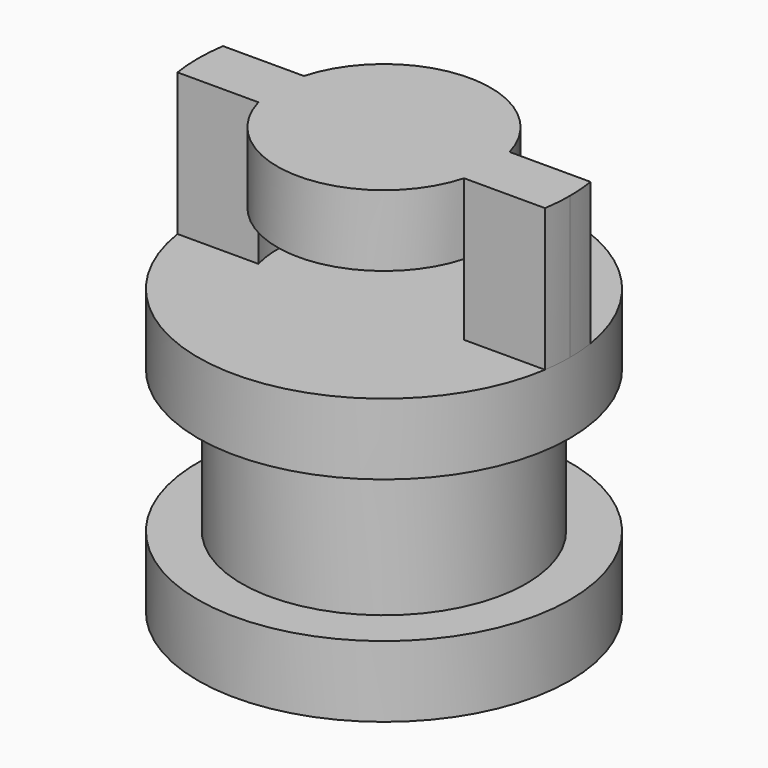
from build123d import *
from build123d import SkipClean  # not in build123d's __all__

# Parameters (mm, degrees)
F0_R      = 4.15
F1_DEPTH  = 1.5875
F3_R      = 4.15
F4_DEPTH  = 1.5875
F6_R      = 2.38125
F7_DEPTH  = 1.5875
F9_DEPTH  = 3.175
F10_R     = 3.175
F11_DEPTH = 3.175
F12_R     = 1.524
F13_DEPTH = 5.159375


# Not quite as in the source:
# - after a boolean that leaves OpenCascade's solid faulty, fix() repairs it


with BuildPart() as f1:
    # F0 (on Top) → F1 (new body)
    with BuildSketch(Plane.XY):
        Circle(F0_R)
    extrude(amount=F1_DEPTH)



with BuildPart() as f4:
    # F3 (on offset) → F4 (new body)
    with BuildSketch(Plane.XY.offset(6.35)):
        Circle(F3_R)
    extrude(amount=-F4_DEPTH)



with BuildPart() as f7:
    # F6 (on offset) → F7 (new body)
    with BuildSketch(Plane.XY.offset(7.9375)):
        Circle(F6_R)
    extrude(amount=F7_DEPTH)


with BuildPart() as f4_1:
    add(f4.part, clean=False)

    add(f7.part)  # F9 merges F7
    # F8 (on face) → F9 (join, through all)
    with BuildSketch(Plane.XY.offset(6.35)):
        with BuildLine():
            Line((2.2950221268, -0.635), (4.1011309416, -0.635))
            ThreePointArc((4.1011309416, -0.635), (4.1377646989, -0.3184388422), (4.15, 0))
            ThreePointArc((4.15, 0), (4.1377646989, 0.3184388422), (4.1011309416, 0.635))
            Line((4.1011309416, 0.635), (2.2950221268, 0.635))
            ThreePointArc((2.2950221268, 0.635), (2.38125, 0), (2.2950221268, -0.635))
        make_face()
        with BuildLine():
            ThreePointArc((-4.1011309416, 0.635), (-4.15, 0), (-4.1011309416, -0.635))
            Line((-4.1011309416, -0.635), (-2.2950221268, -0.635))
            ThreePointArc((-2.2950221268, -0.635), (-2.38125, 0), (-2.2950221268, 0.635))
            Line((-2.2950221268, 0.635), (-4.1011309416, 0.635))
        make_face()
    extrude(amount=F9_DEPTH)

    add(f4_1.part.fix(), mode=Mode.REPLACE)


with BuildPart() as f1_1:
    add(f1.part, clean=False)

    add(f4_1.part)  # F11 merges F4
    # F10 (on face) → F11 (join, through all)
    with BuildSketch(Plane.XY.offset(1.5875)):
        Circle(F10_R)
    extrude(amount=F11_DEPTH)

    # F12 (on face) → F13 (cut)
    with BuildSketch(Plane(origin=(0, 0, 0), x_dir=(1, 0, 0), z_dir=(0, 0, -1))):
        Circle(F12_R)
    with SkipClean():  # cleaning this boolean's faces spoils the solid; the shape is the same uncleaned
        extrude(amount=-F13_DEPTH, mode=Mode.SUBTRACT)


solid = f1_1.part
